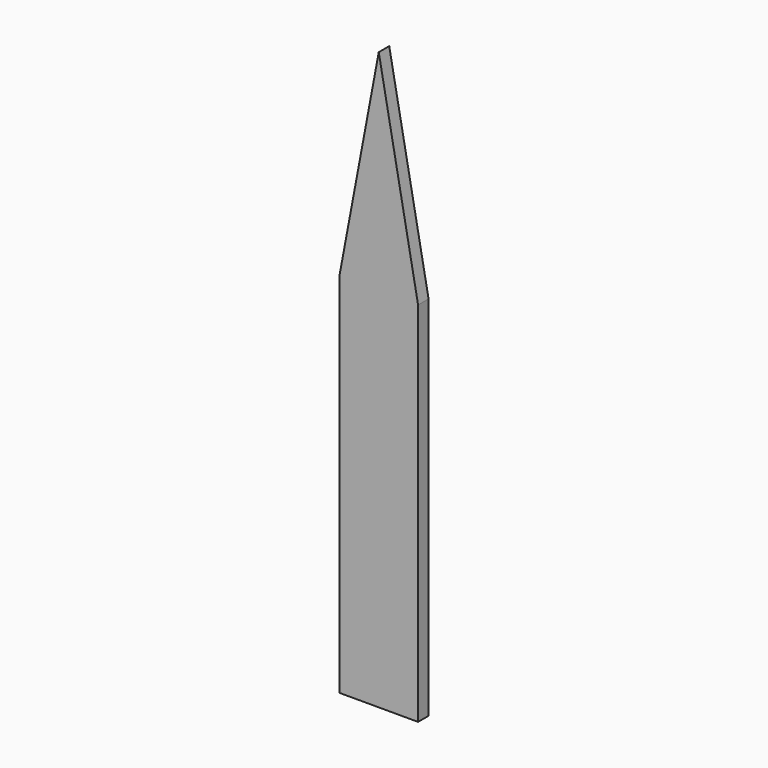
from build123d import *

# Parameters (mm, degrees)
F1_DEPTH = 3.175
F3_DEPTH = 25.4


# Not quite as in the source:
# - a length typed as a fraction of an inch, garbled in the dataset ("3 / 203.2 mm" for 3/8 in), is restored


with BuildPart() as f1:
    # F0 (on Front) → F1 (new body)
    with BuildSketch(Plane.XZ):
        Polygon((0, 88.9), (0, 0), (19.05, 0), (19.05, 88.9), (9.525, 139.7), align=None)
        Polygon((0, 139.7), (0, 88.9), (9.525, 139.7), align=None)
        Polygon((9.525, 139.7), (19.05, 88.9), (19.05, 139.7), align=None)
    extrude(amount=F1_DEPTH)

    # F2 (on face) → F3 (cut)
    with BuildSketch(Plane.XZ.offset(3.175)):
        Polygon((0, 139.7), (0, 88.9), (9.525, 139.7), align=None)
        Polygon((19.05, 139.7), (9.525, 139.7), (19.05, 88.9), align=None)
    extrude(amount=-F3_DEPTH, mode=Mode.SUBTRACT)


solid = f1.part
